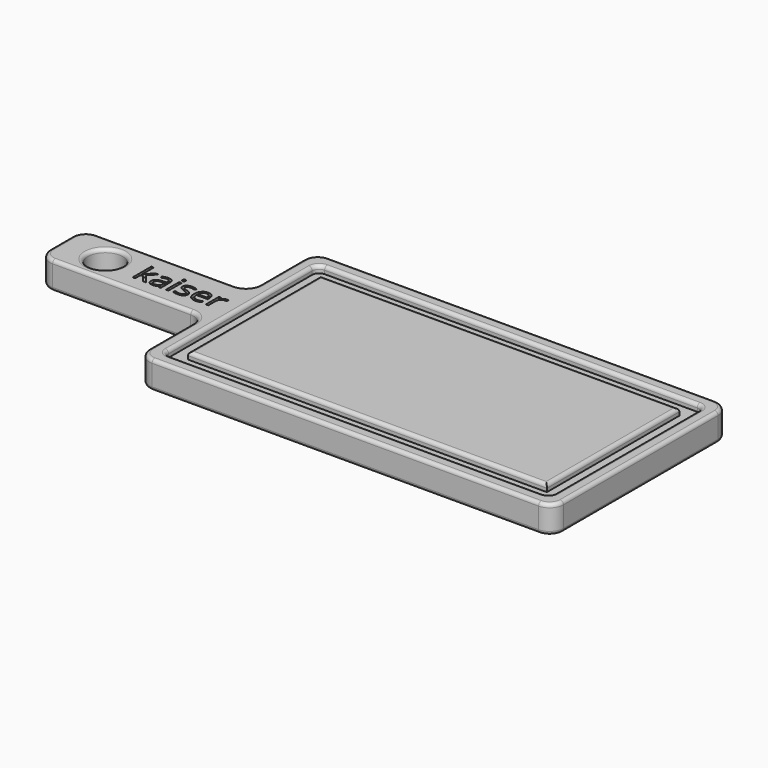
from build123d import *

# Parameters (mm, degrees)
F0_W          = 152.4
F0_H          = 50.8
F1_DEPTH      = 25.4
F2_R          = 15.875
F3_DEPTH      = 25.4
F5_DEPTH      = 6.35
F6_R          = 6.35
F7_R          = 12.7
F8_R          = 12.7
F9_R          = 3.175
F10_TEXT_SIZE = 28.3861443941
F11_DEPTH     = 2.54


# Not quite as in the source:
# - Text() gives the source's letters only with a copy of the font that has no kerning and outlines rounded to 1/6400 em; it was checked with that copy


with BuildPart() as f1:
    # F0 (on Top) → F1 (new body)
    with BuildSketch(Plane.XY):
        Polygon((0, 76.2), (0, 0), (381, 0), (381, 203.2), (0, 203.2), (0, 127), align=None)
        with Locations((-76.2, 101.6)):
            Rectangle(F0_W, F0_H)
    extrude(amount=F1_DEPTH)

    # F2 (on face) → F3 (cut)
    with BuildSketch(Plane.XY.offset(25.4)):
        with Locations((-111.1298849044, 100.965)):
            Circle(F2_R)
    extrude(amount=-F3_DEPTH, mode=Mode.SUBTRACT)

    # F4 (on face) → F5 (cut)
    with BuildSketch(Plane.XY.offset(25.4)):
        Polygon((12.7, 190.5), (12.7, 127), (12.7, 76.2), (12.7, 12.7), (368.3, 12.7), (368.3, 190.5), align=None)
        Polygon((25.4, 76.2), (25.4, 127), (25.4, 177.8), (355.6, 177.8), (355.6, 25.4), (25.4, 25.4), align=None, mode=Mode.SUBTRACT)
    extrude(amount=-F5_DEPTH, mode=Mode.SUBTRACT)

    # F6
    f6_edges = [f1.edges().sort_by_distance(p)[0] for p in [
        (12.7, 190.5, 22.225),
        (368.3, 190.5, 22.225),
        (12.7, 12.7, 22.225),
        (368.3, 12.7, 22.225),
    ]]
    fillet(f6_edges, radius=F6_R)

    # F7
    f7_edges = [f1.edges().sort_by_distance(p)[0] for p in [
        (381, 203.2, 12.7),
        (0, 203.2, 12.7),
        (0, 0, 12.7),
        (381, 0, 12.7),
    ]]
    fillet(f7_edges, radius=F7_R)

    # F8
    f8_edges = [f1.edges().sort_by_distance(p)[0] for p in [
        (0, 127, 12.7),
        (-152.4, 127, 12.7),
        (-152.4, 76.2, 12.7),
        (0, 76.2, 12.7),
    ]]
    fillet(f8_edges, radius=F8_R)

    # F9
    f9_edges = [f1.edges().sort_by_distance(p)[0] for p in [
        (190.5, 177.8, 25.4),
        (355.6, 101.6, 25.4),
        (190.5, 25.4, 25.4),
        (25.4, 101.6, 25.4),
        (0, 38.1, 25.4),
        (-3.719744, 72.480256, 25.4),
        (3.719744, 3.719744, 25.4),
        (-76.2, 76.2, 25.4),
        (190.5, 0, 25.4),
        (-148.680256, 79.919744, 25.4),
        (377.280256, 3.719744, 25.4),
        (-152.4, 101.6, 25.4),
        (381, 101.6, 25.4),
        (-148.680256, 123.280256, 25.4),
        (377.280256, 199.480256, 25.4),
        (-76.2, 127, 25.4),
        (190.5, 203.2, 25.4),
        (-3.719744, 130.719744, 25.4),
        (3.719744, 199.480256, 25.4),
        (0, 165.1, 25.4),
        (190.5, 12.7, 25.4),
        (14.559872, 14.559872, 25.4),
        (366.440128, 14.559872, 25.4),
        (12.7, 101.6, 25.4),
        (368.3, 101.6, 25.4),
        (14.559872, 188.640128, 25.4),
        (366.440128, 188.640128, 25.4),
        (190.5, 190.5, 25.4),
        (-127.004885, 100.965, 25.4),
        (0, 38.1, 0),
        (-3.719744, 72.480256, 0),
        (3.719744, 3.719744, 0),
        (-76.2, 76.2, 0),
        (190.5, 0, 0),
        (-148.680256, 79.919744, 0),
        (377.280256, 3.719744, 0),
        (-152.4, 101.6, 0),
        (381, 101.6, 0),
        (-148.680256, 123.280256, 0),
        (377.280256, 199.480256, 0),
        (-76.2, 127, 0),
        (190.5, 203.2, 0),
        (-3.719744, 130.719744, 0),
        (3.719744, 199.480256, 0),
        (0, 165.1, 0),
        (-127.004885, 100.965, 0),
    ]]
    fillet(f9_edges, radius=F9_R)

    # F10 (on face) → F11 (cut)
    with BuildSketch(Plane.XY.offset(25.4)):
        with Locations((-80.3594006456, 90.8375647935)):
            Text('kaiser', F10_TEXT_SIZE, font='Open Sans', text_align=(TextAlign.LEFT, TextAlign.BOTTOM))
    extrude(amount=-F11_DEPTH, mode=Mode.SUBTRACT)


solid = f1.part
